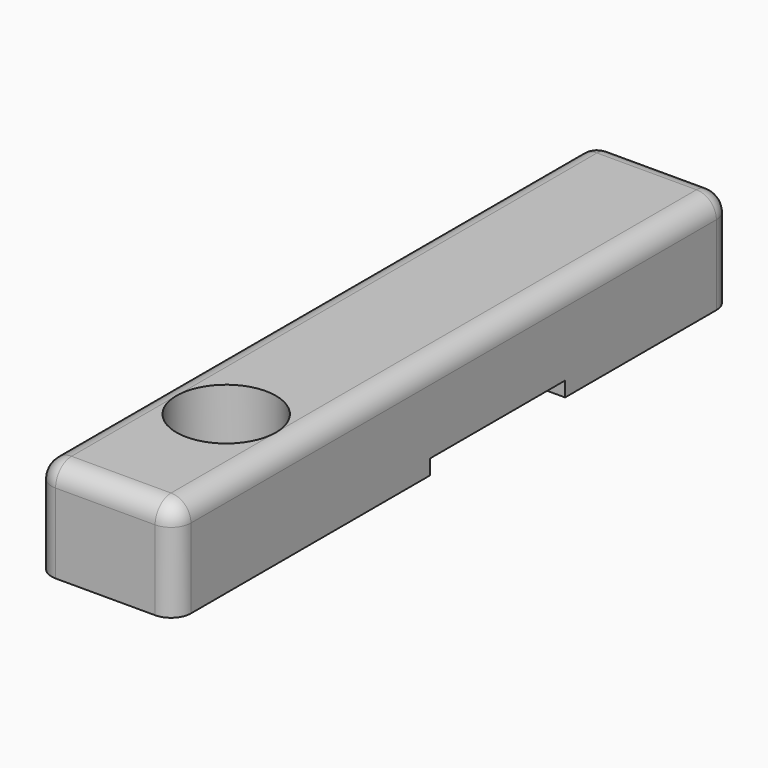
from build123d import *

# Parameters (mm, degrees)
F1_DEPTH = 7
F2_R     = 2.5
F3_DEPTH = 5.001
F4_R     = 0.99999


# Not quite as in the source:
# - a fillet or chamfer is up to 0.001 mm smaller than in the source, because OpenCascade refuses the exact size


with BuildPart() as f1:
    # F0 (on Right) → F1 (new body)
    with BuildSketch(Plane.YZ):
        Polygon((35, 0), (0, 0), (0, -5), (16, -5), (16, -4.25), (24.5, -4.25), (24.5, -5), (35, -5), align=None)
    extrude(amount=-F1_DEPTH)

    # F2 (on face) → F3 (cut, through all)
    with BuildSketch(Plane.XY):
        with Locations((-3.5, 7.5868815184)):
            Circle(F2_R)
    extrude(amount=-F3_DEPTH, mode=Mode.SUBTRACT)

    # F4 (radius 1 in the source; OpenCascade refuses exactly that, so slightly less here)
    f4_edges = [f1.edges().sort_by_distance(p)[0] for p in [
        (-3.5, 35, 0),
        (-7, 17.5, 0),
        (-3.5, 0, 0),
        (0, 17.5, 0),
        (0, 0, -2.5),
        (0, 35, -2.5),
        (-7, 35, -2.5),
        (-7, 0, -2.5),
    ]]
    fillet(f4_edges, radius=F4_R)


solid = f1.part
